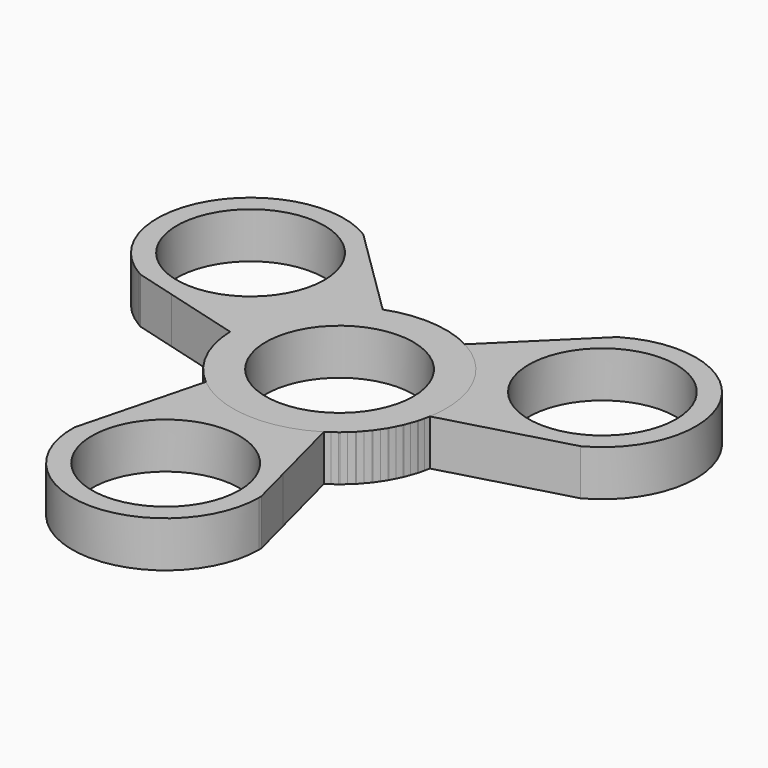
from build123d import *

# Parameters (mm, degrees)
F0_R     = 16.25
F0_R_2   = 11.25
F2_DEPTH = 7
F1_R     = 11.25
F3_DEPTH = 7
F4_COUNT = 3


# Not quite as in the source:
# - a feature names something its author has since deleted; it is built from what else it names


with BuildPart() as f2:
    # F0 (on Top) → F2 (new body)
    with BuildSketch(Plane.XY):
        with Locations((-36.4034558124, 12.0280578335)):
            Circle(F0_R)
        with Locations((-36.4034558124, 12.0280578335)):
            Circle(F0_R_2, mode=Mode.SUBTRACT)
    extrude(amount=F2_DEPTH)

    # F1 (on face) → F3 (join)
    with BuildSketch(Plane.XY):
        with BuildLine():
            ThreePointArc((-51.7026241701, -19.3605581831), (-37.683132397, -34.0557455005), (-23.2096348578, -19.8074982803))
            ThreePointArc((-23.2096348578, -19.8074982803), (-23.2113876375, -19.584000741), (-23.2166455455, -19.3605581831))
            Line((-23.2166455455, -19.3605581831), (-24.7919850828, -13.2811555695))
            ThreePointArc((-24.7919850828, -13.2811555695), (-37.4596348578, -5.5574982803), (-50.1272846328, -13.2811555695))
            Line((-50.1272846328, -13.2811555695), (-51.7026241701, -19.3605581831))
        make_face()
        with Locations((-37.4596348578, -19.8074982803)):
            Circle(F1_R, mode=Mode.SUBTRACT)
        with BuildLine():
            ThreePointArc((-50.1272846328, -13.2811555695), (-37.4596348578, -5.5574982803), (-24.7919850828, -13.2811555695))
            Line((-24.7919850828, -13.2811555695), (-27.7811233105, -1.7457536298))
            ThreePointArc((-27.7811233105, -1.7457536298), (-37.5015275941, -4.1847993595), (-46.8042843024, -0.4573443115))
            Line((-46.8042843024, -0.4573443115), (-50.1272846328, -13.2811555695))
        make_face()
    extrude(amount=F3_DEPTH)


with BuildPart() as f4_1:
    # F4: instance of F2
    add(f2.part.rotate(Axis((-36.4034558124, 12.0280578335, 0), (0, 0, 1)), 1 * 360 / F4_COUNT))


with BuildPart() as f4_2:
    # F4: instance of F2
    add(f2.part.rotate(Axis((-36.4034558124, 12.0280578335, 0), (0, 0, 1)), 2 * 360 / F4_COUNT))


solid = Compound([f2.part, f4_1.part, f4_2.part])
